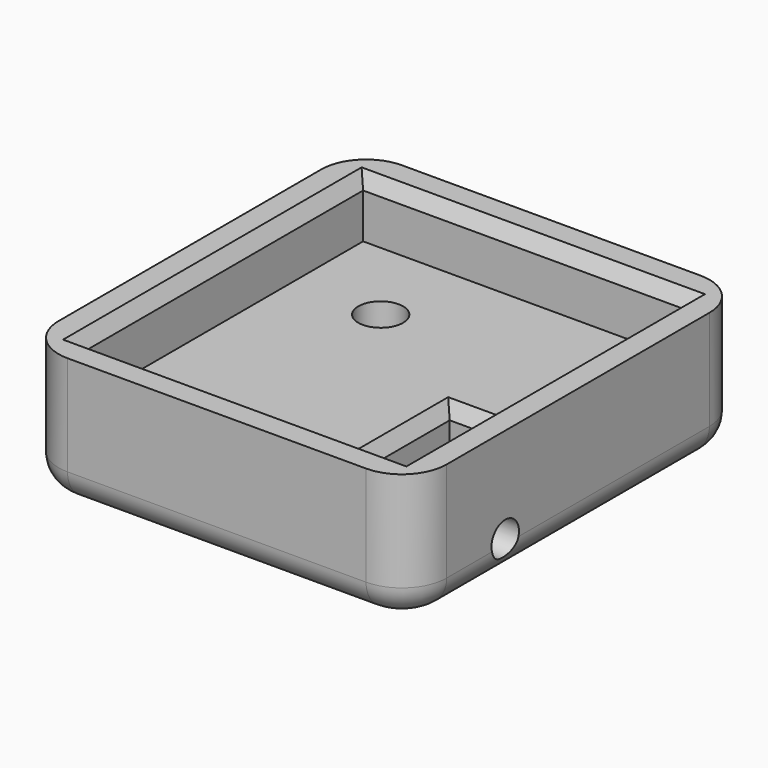
from build123d import *

# Parameters (mm, degrees)
F0_W       = 22
F0_H       = 2
F0_R       = 1.5
F1_DEPTH   = 4.7
F2_DEPTH   = 8.7
F3_R       = 1.5
F4_DEPTH   = 4.701
F6_SIZE2   = 1
F6_SIZE    = 0.5
F6_2_SIZE2 = 1
F6_2_SIZE  = 0.5
F6_3_SIZE2 = 1
F6_3_SIZE  = 0.5
F7_R       = 3
F8_R       = 1.99999
F5_R       = 1.15
F9_DEPTH   = 26.0010001


# Not quite as in the source:
# - a fillet or chamfer is up to 0.001 mm smaller than in the source, because OpenCascade refuses the exact size


with BuildPart() as f1:
    # F0 (on Top) → F1 (new body)
    with BuildSketch(Plane.XY):
        with Locations((0, 12.5)):
            Rectangle(F0_W, F0_H)
        Polygon((-11, -12.5), (-11, 11.5), (-11, 13.5), (-13, 13.5), (-13, -14.5), (-11, -14.5), align=None)
        Polygon((11, 13.5), (11, 11.5), (11, -12.5), (11, -14.5), (13, -14.5), (13, 13.5), align=None)
        Polygon((4, -12.5), (-11, -12.5), (-11, -14.5), (11, -14.5), (11, -12.5), (6.7, -12.5), align=None)
        Polygon((11, 11.5), (-11, 11.5), (-11, -12.5), (4, -12.5), (4, 0), (6.7, 0), (6.7, -12.5), (11, -12.5), align=None)
        with Locations((-5.1, 5.6)):
            Circle(F0_R, mode=Mode.SUBTRACT)
    extrude(amount=F1_DEPTH)

    # F0 (on Top) → F2 (join)
    with BuildSketch(Plane.XY):
        Polygon((11, 13.5), (11, 11.5), (11, -12.5), (11, -14.5), (13, -14.5), (13, 13.5), align=None)
        Polygon((4, -12.5), (-11, -12.5), (-11, -14.5), (11, -14.5), (11, -12.5), (6.7, -12.5), align=None)
        Polygon((-11, -12.5), (-11, 11.5), (-11, 13.5), (-13, 13.5), (-13, -14.5), (-11, -14.5), align=None)
        with Locations((0, 12.5)):
            Rectangle(F0_W, F0_H)
    extrude(amount=F2_DEPTH)

    # F3 (on face) → F4 (cut, through all)
    with BuildSketch(Plane.XY.offset(4.7)):
        with Locations((-5.1, 5.6)):
            Circle(F3_R)
    extrude(amount=-F4_DEPTH, mode=Mode.SUBTRACT)

    # F6
    f6_edges = [f1.edges().sort_by_distance(p)[0] for p in [
        (0, 11.5, 8.7),
        (11, -0.5, 8.7),
        (-11, -0.5, 8.7),
        (0, -12.5, 8.7),
    ]]
    f6_side = f1.faces().sort_by_distance((11.382099, -0.5, 8.7))[0]
    chamfer(f6_edges, length=F6_SIZE, length2=F6_SIZE2, reference=f6_side)

    # F6#2
    f6_2_edges = [f1.edges().sort_by_distance(p)[0] for p in [
        (-6.6, 5.6, 0),
    ]]
    f6_2_side = f1.faces().sort_by_distance((-0.210298, -0.280343, 0))[0]
    chamfer(f6_2_edges, length=F6_2_SIZE, length2=F6_2_SIZE2, reference=f6_2_side)

    # F6#3
    f6_3_edges = [f1.edges().sort_by_distance(p)[0] for p in [
        (5.35, 0, 4.7),
        (4, -6.25, 4.7),
    ]]
    f6_3_side = f1.faces().sort_by_distance((-0.29663, -0.190169, 4.7))[0]
    chamfer(f6_3_edges, length=F6_3_SIZE, length2=F6_3_SIZE2, reference=f6_3_side)

    # F7
    f7_edges = [f1.edges().sort_by_distance(p)[0] for p in [
        (-13, -14.5, 4.35),
        (13, -14.5, 4.35),
        (-13, 13.5, 4.35),
        (13, 13.5, 4.35),
    ]]
    fillet(f7_edges, radius=F7_R)

    # F8 (radius 2 in the source; OpenCascade refuses exactly that, so slightly less here)
    f8_edges = [f1.edges().sort_by_distance(p)[0] for p in [
        (13, -0.5, 0),
        (12.12132, -13.62132, 0),
        (0, -14.5, 0),
        (-12.12132, -13.62132, 0),
        (12.12132, 12.62132, 0),
        (0, 13.5, 0),
        (-12.12132, 12.62132, 0),
        (-13, -0.5, 0),
    ]]
    fillet(f8_edges, radius=F8_R)

    # F5 (on face) → F9 (cut, through all)
    with BuildSketch(Plane.YZ.offset(13)):
        with Locations((-6.6, 2.3)):
            Circle(F5_R)
    extrude(amount=-F9_DEPTH, mode=Mode.SUBTRACT)


solid = f1.part
